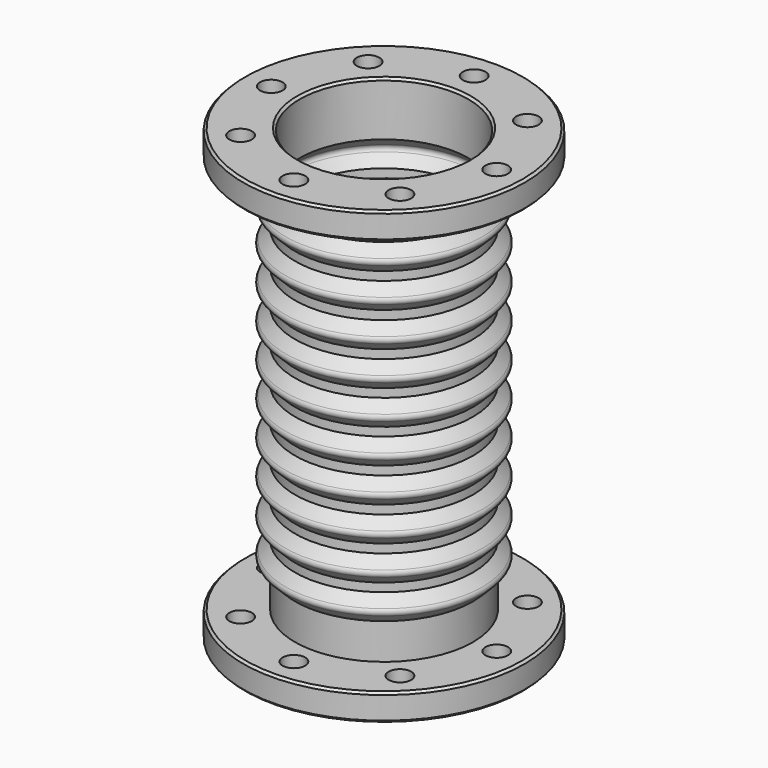
from build123d import *

# Parameters (mm, degrees)
F3_D     = 10
F3_DEPTH = 20
F3_TIP   = 3.0043030951
F5_D     = 10
F5_DEPTH = 12
F5_TIP   = 3.0043030951
F6_SIZE  = 1


# Not quite as in the source:
# - ends of sketch curves that miss each other by under 0.0002 mm in the source are joined
# - a feature names something its author has since deleted; it is built from what else it names


with BuildPart() as f1:
    # F0 (on Front) → F1 (revolve)
    with BuildSketch(Plane.XZ):
        Polygon((37.5, 200), (37.5, 188), (39.5, 188), (49.1224490106, 188), (62.5, 188), (62.5, 200), align=None)
        Polygon((37.5, 12), (37.5, 0), (62.5, 0), (62.5, 12), (39.5, 12), align=None)
        with BuildLine():
            Line((37.5, 24), (37.5, 12))
            Line((37.5, 12), (39.5, 12))
            Line((39.5, 12), (39.5, 24))
            Line((39.5, 24), (39.5, 27.8862919658))
            Line((39.5, 27.8862919658), (43.7426406871, 32.128932653))
            ThreePointArc((43.7426406871, 32.128932653), (44.3284271247, 33.5431462153), (43.7426406871, 34.9573597777))
            Line((43.7426406871, 34.9573597777), (39.5, 39.2000004648))
            Line((39.5, 39.2000004648), (39.5, 42.9784080237))
            Line((39.5, 42.9784080237), (43.7498388975, 47.2282469212))
            ThreePointArc((43.7498388975, 47.2282469212), (44.3356188252, 48.6373576102), (43.7570370141, 50.0494391041))
            Line((43.7570370141, 50.0494391041), (39.5, 54.350145626))
            Line((39.5, 54.350145626), (39.5, 58.236437127))
            Line((39.5, 58.236437127), (43.7438828615, 62.4803199885))
            ThreePointArc((43.7438828615, 62.4803199885), (44.329669106, 63.8936548151), (43.7451250353, 65.3075038473))
            Line((43.7451250353, 65.3075038473), (39.5, 69.5600961327))
            Line((39.5, 69.5600961327), (39.5, 73.4463876337))
            Line((39.5, 73.4463876337), (43.7488831793, 77.695270813))
            ThreePointArc((43.7488831793, 77.695270813), (44.3346647243, 79.1050605139), (43.7551256104, 80.5174278297))
            Line((43.7551256104, 80.5174278297), (39.5, 84.8103691815))
            Line((39.5, 84.8103691815), (39.5, 88.6966606826))
            Line((39.5, 88.6966606826), (43.7426406871, 92.9393013697))
            ThreePointArc((43.7426406871, 92.9393013697), (44.3284271247, 94.3535149321), (43.7426406871, 95.7677284944))
            Line((43.7426406871, 95.7677284944), (39.5, 100.0103691815))
            Line((39.5, 100.0103691815), (39.4999985099, 103.8227102011))
            Line((39.4999985099, 103.8227102011), (43.742639197, 108.0653508883))
            ThreePointArc((43.742639197, 108.0653508883), (44.3284256346, 109.4795644506), (43.742639197, 110.893778013))
            Line((43.742639197, 110.893778013), (39.4999985099, 115.1364187001))
            Line((39.4999985099, 115.1364187001), (39.5, 118.9536920041))
            Line((39.5, 118.9536920041), (43.7434366066, 123.1971286107))
            ThreePointArc((43.7434366066, 123.1971286107), (44.329222965, 124.6107792146), (43.744232526, 126.0247593679))
            Line((43.744232526, 126.0247593679), (39.4999985099, 130.2737747311))
            Line((39.4999985099, 130.2737747311), (39.4999985099, 134.1600662321))
            Line((39.4999985099, 134.1600662321), (43.7315679123, 138.3916356345))
            ThreePointArc((43.7315679123, 138.3916356345), (44.3173391477, 139.8136471942), (43.7204969642, 141.2310477108))
            Line((43.7204969642, 141.2310477108), (39.4431017339, 145.4422473907))
            Line((39.4431017339, 145.4422473907), (39.4431017339, 149.4444662482))
            Line((39.4431017339, 149.4444662482), (43.742639197, 153.7440037112))
            ThreePointArc((43.742639197, 153.7440037112), (44.3284256346, 155.1582172736), (43.742639197, 156.572430836))
            Line((43.742639197, 156.572430836), (39.4999985099, 160.8150715231))
            Line((39.4999985099, 160.8150715231), (39.4999985099, 164.6862919658))
            Line((39.4999985099, 164.6862919658), (43.7426393252, 168.9289327811))
            ThreePointArc((43.7426393252, 168.9289327811), (44.3284257628, 170.3431462529), (43.7426394533, 171.7573597777))
            Line((43.7426394533, 171.7573597777), (39.5, 176))
            Line((39.5, 176), (39.5, 188))
            Line((39.5, 188), (37.5, 188))
            Line((37.5, 188), (37.5, 176.03901124))
            Line((37.5, 176.03901124), (41.7426406871, 171.7963705529))
            ThreePointArc((41.7426406871, 171.7963705529), (42.3284271247, 170.3821569905), (41.7426406871, 168.9679434281))
            Line((41.7426406871, 168.9679434281), (37.5, 164.725302741))
            Line((37.5, 164.725302741), (37.5, 160.8540822983))
            Line((37.5, 160.8540822983), (41.7426406871, 156.6114416112))
            ThreePointArc((41.7426406871, 156.6114416112), (42.3284271247, 155.1972280488), (41.7426406871, 153.7830144864))
            Line((41.7426406871, 153.7830144864), (37.5, 149.5403737993))
            Line((37.5, 149.5403737993), (37.5, 145.5127855062))
            Line((37.5, 145.5127855062), (41.7426406871, 141.2701448191))
            ThreePointArc((41.7426406871, 141.2701448191), (42.3284271247, 139.8559312568), (41.7426406871, 138.4417176944))
            Line((41.7426406871, 138.4417176944), (37.5, 134.1990770073))
            Line((37.5, 134.1990770073), (37.5000014901, 130.3064112782))
            Line((37.5000014901, 130.3064112782), (41.7426421772, 126.0637705911))
            ThreePointArc((41.7426421772, 126.0637705911), (42.3284286149, 124.6495570288), (41.7426421772, 123.2353434664))
            Line((41.7426421772, 123.2353434664), (37.5000014901, 118.9927027793))
            Line((37.5000014901, 118.9927027793), (37.5000014901, 115.1364182353))
            Line((37.5000014901, 115.1364182353), (41.7426406871, 110.8937775482))
            ThreePointArc((41.7426406871, 110.8937775482), (42.3284271247, 109.4795639858), (41.7426406871, 108.0653504234))
            Line((41.7426406871, 108.0653504234), (37.5, 103.8227097363))
            Line((37.5, 103.8227097363), (37.5000014901, 100.0103687167))
            Line((37.5000014901, 100.0103687167), (41.7426421772, 95.7677280296))
            ThreePointArc((41.7426421772, 95.7677280296), (42.3284286149, 94.3535144672), (41.7426421772, 92.9393009049))
            Line((41.7426421772, 92.9393009049), (37.5000014901, 88.6966602177))
            Line((37.5000014901, 88.6966602177), (37.5000014901, 84.8103687167))
            Line((37.5000014901, 84.8103687167), (41.7551271005, 80.5174273649))
            ThreePointArc((41.7551271005, 80.5174273649), (42.3346662144, 79.1050600491), (41.7488846694, 77.6952703481))
            Line((41.7488846694, 77.6952703481), (37.5000014901, 73.4463871689))
            Line((37.5000014901, 73.4463871689), (37.5000014901, 69.5600956678))
            Line((37.5000014901, 69.5600956678), (41.7451265254, 65.3075033825))
            ThreePointArc((41.7451265254, 65.3075033825), (42.3296705962, 63.8936543503), (41.7438843516, 62.4803195236))
            Line((41.7438843516, 62.4803195236), (37.5000014901, 58.2364366622))
            Line((37.5000014901, 58.2364366622), (37.5000014901, 54.3501451612))
            Line((37.5000014901, 54.3501451612), (41.7570385042, 50.0494386393))
            ThreePointArc((41.7570385042, 50.0494386393), (42.3356203154, 48.6373571454), (41.7498403876, 47.2282464563))
            Line((41.7498403876, 47.2282464563), (37.5000014901, 42.9784075589))
            Line((37.5000014901, 42.9784075589), (37.5000014901, 39.2))
            Line((37.5000014901, 39.2), (41.7426421772, 34.9573593129))
            ThreePointArc((41.7426421772, 34.9573593129), (42.3284286149, 33.5431457505), (41.7426421772, 32.1289321881))
            Line((41.7426421772, 32.1289321881), (37.5000014901, 27.886291501))
            Line((37.5000014901, 27.886291501), (37.5, 24))
        make_face()
    revolve(axis=Axis((0, 0, 100), (0, 0, 1)))

    # F3
    with Locations(Plane.XY.offset(200)):
        with Locations((-50, 0), (-35.3553390593, 35.3553390593), (0, 50), (35.3553390593, 35.3553390593), (50, 0), (35.3553390593, -35.3553390593), (0, -50), (-35.3553390593, -35.3553390593)):
            Hole(F3_D / 2, depth=F3_DEPTH)
            with Locations((0, 0, -(F3_DEPTH + F3_TIP / 2))):  # 118° drill point
                Cone(0, F3_D / 2, F3_TIP, mode=Mode.SUBTRACT)

    # F5
    with Locations(Plane(origin=(0, 0, 0), x_dir=(1, 0, 0), z_dir=(0, 0, -1))):
        with Locations((0.1593066842, -49.8268464117), (-35.1960323751, -35.1821854711), (-49.8406933158, 0.1731535883), (-35.1960323751, 35.5284926476), (0.1593066842, 50.1731535883), (35.5146457436, 35.5284926476), (50.1593066842, 0.1731535883), (35.5146457436, -35.1821854711)):
            Hole(F5_D / 2, depth=F5_DEPTH)
            with Locations((0, 0, -(F5_DEPTH + F5_TIP / 2))):  # 118° drill point
                Cone(0, F5_D / 2, F5_TIP, mode=Mode.SUBTRACT)

    # F6
    f6_edges = [f1.edges().sort_by_distance(p)[0] for p in [
        (-62.5, 0, 200),
        (-37.5, 0, 200),
        (-62.5, 0, 188),
        (-62.5, 0, 12),
        (-62.5, 0, 0),
    ]]
    chamfer(f6_edges, length=F6_SIZE)


solid = f1.part
